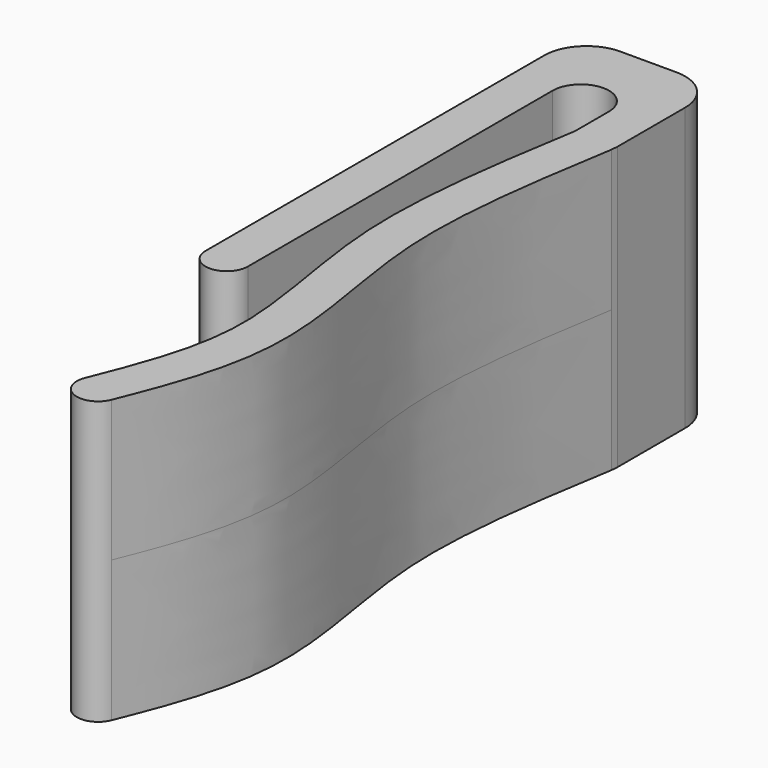
from build123d import *

# Parameters (mm, degrees)
F1_DEPTH = 10


# Not quite as in the source:
# - the dataset's text gives a spline's control points without its knots; the knots are read off the source's solid


with BuildPart() as f1:
    # F0 (on Top) → F1 (new body, symmetric)
    with BuildSketch(Plane.XY):
        with BuildLine():
            ThreePointArc((-9.0035215598, 20.6597696395), (-11.1248419033, 19.7810899831), (-12.0035215598, 17.6597696395))
            Line((-12.0035215598, 17.6597696395), (-12.0035215598, -12.3402303605))
            ThreePointArc((-12.0035215598, -12.3402303605), (-10.5035215598, -13.8402303605), (-9.0035215598, -12.3402303605))
            Line((-9.0035215598, -12.3402303605), (-9.0035215598, 14.6597696395))
            ThreePointArc((-9.0035215598, 14.6597696395), (-7.0035215598, 16.6597696395), (-5.0035215598, 14.6597696395))
            Line((-5.0035215598, 14.6597696395), (-5.0035215598, 11.6597696395))
            add(Edge.make_bspline(
                [(-5.0035215598, 11.6597696395), (-5.9307724886, 5.934399773), (-7.683272066, -4.8865203894), (-3.6772391277, -18.3264952053), (-6.4230985269, -25.2014576829), (-7.7084186487, -28.4195858985)],
                knots=[0, 0, 0, 0, 0.3740809379, 0.7070110854, 1, 1, 1, 1], degree=3))
            ThreePointArc((-7.7084186487, -28.4195858985), (-6.8717808793, -30.3689542726), (-4.9224125052, -29.5323165033))
            add(Edge.make_bspline(
                [(-2.0421082014, 11.1801546363), (-2.3519512176, 9.2670092157), (-2.810720014, 6.4312344897), (-3.2713607988, 2.7649872941), (-3.4691384037, 0.5327621954), (-3.5578713082, -1.2105065224), (-3.5860914841, -2.495070727), (-3.5748148513, -3.5447149712), (-3.5432481695, -4.371998696), (-3.4963004463, -5.1879592247), (-3.4065553568, -6.2079792032), (-3.2085671451, -7.8568119023), (-2.8847333006, -9.9401893948), (-2.4630204194, -12.4768023811), (-2.1674909882, -14.6258210905), (-2.0230521201, -16.3739271894), (-1.9854344258, -17.4798061875), (-1.9961827402, -18.3738801735), (-2.0379493463, -19.2708103603), (-2.1453912364, -20.3631681654), (-2.3501563661, -21.6351730435), (-2.7078547349, -23.2768631773), (-3.283043942, -25.2319910338), (-4.0880236454, -27.443865427), (-4.6482297509, -28.8458297338), (-4.9224125052, -29.5323165033)],
                knots=[0, 0, 0, 0, 0.125, 0.1875, 0.25, 0.28125, 0.3125, 0.34375, 0.359375, 0.375, 0.40625, 0.4375, 0.5, 0.5625, 0.625, 0.65625, 0.6875, 0.703125, 0.71875, 0.75, 0.78125, 0.8125, 0.875, 0.9375, 1, 1, 1, 1], degree=3))
            Line((-2.0421082014, 11.1801546363), (-2.0035215598, 11.6597696395))
            Line((-2.0035215598, 11.6597696395), (-2.0035215598, 14.6597696395))
            Line((-2.0035215598, 14.6597696395), (-2.0035215598, 17.6597696395))
            ThreePointArc((-2.0035215598, 17.6597696395), (-2.8822012162, 19.7810899831), (-5.0035215598, 20.6597696395))
            Line((-5.0035215598, 20.6597696395), (-9.0035215598, 20.6597696395))
        make_face()
    extrude(amount=F1_DEPTH, both=True)


solid = f1.part
